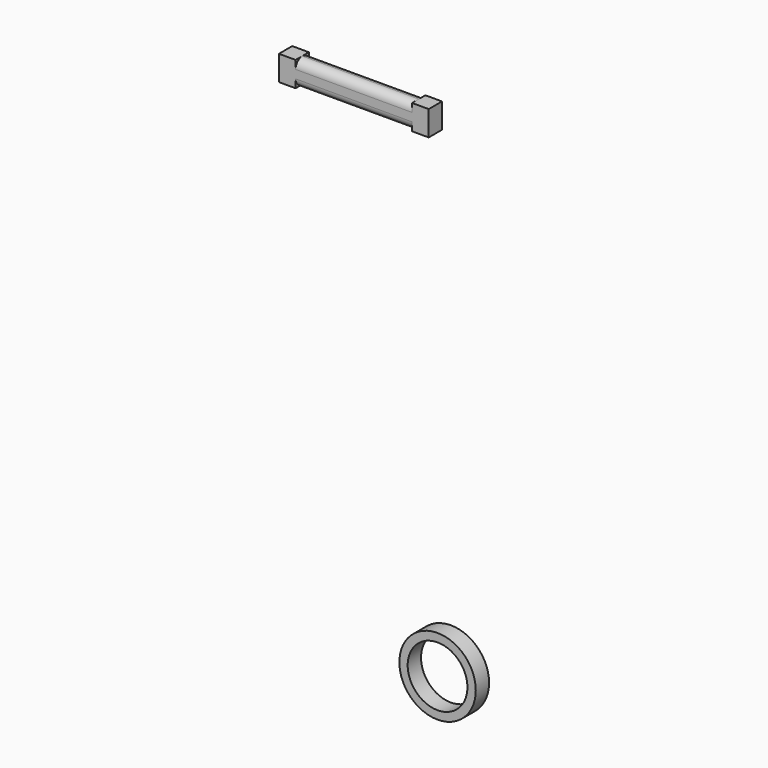
from build123d import *

# Parameters (mm, degrees)
F0_W     = 14
F0_H     = 3
F1_DEPTH = 2
F4_R     = 0.99999
F2_W     = 2
F2_H     = 3
F5_DEPTH = 2
F3_W     = 2
F3_H     = 3
F6_DEPTH = 2
F7_R     = 4.59
F7_R_2   = 3.59
F8_DEPTH = 2


# Not quite as in the source:
# - a fillet or chamfer is up to 0.001 mm smaller than in the source, because OpenCascade refuses the exact size


with BuildPart() as f1:
    # F0 (on Front) → F1 (new body)
    with BuildSketch(Plane.XZ):
        with Locations((-36.3600781634, 30.342812404)):
            Rectangle(F0_W, F0_H)
    extrude(amount=F1_DEPTH)

    # F4 (radius 1 in the source; OpenCascade refuses exactly that, so slightly less here)
    f4_edges = [f1.edges().sort_by_distance(p)[0] for p in [
        (-36.360078, 0, 31.842812),
        (-36.360078, 0, 28.842812),
        (-36.360078, -2, 31.842812),
        (-36.360078, -2, 28.842812),
    ]]
    fillet(f4_edges, radius=F4_R)

    # F2 (on face) → F5 (join)
    with BuildSketch(Plane(origin=(-43.3600781634, 0, 0), x_dir=(0, -1, 0), z_dir=(-1, 0, 0))):
        with Locations((1, 30.342812404)):
            Rectangle(F2_W, F2_H)
    extrude(amount=F5_DEPTH)

    # F3 (on face) → F6 (join)
    with BuildSketch(Plane.YZ.offset(-29.3600781634)):
        with Locations((-1, 30.342812404)):
            Rectangle(F3_W, F3_H)
    extrude(amount=F6_DEPTH)


with BuildPart() as f8:
    # F7 (on Front) → F8 (new body)
    with BuildSketch(Plane.XZ):
        with Locations((-26.2961350381, -27.8185419738)):
            Circle(F7_R)
        with Locations((-26.2961350381, -27.8185419738)):
            Circle(F7_R_2, mode=Mode.SUBTRACT)
    extrude(amount=F8_DEPTH)


solid = Compound([f1.part, f8.part])
